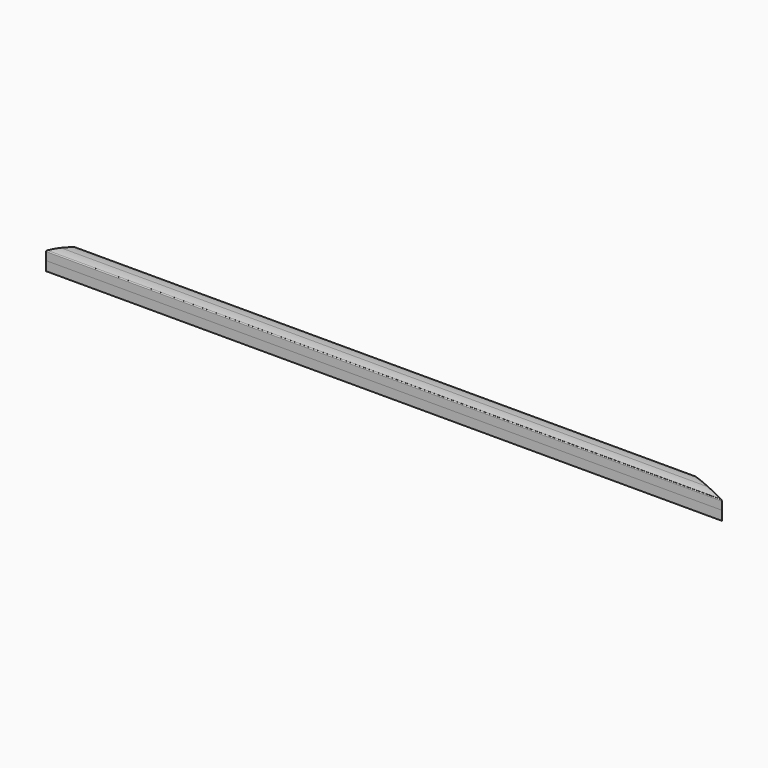
from build123d import *

# Parameters (mm, degrees)
F2_DEPTH      = 1000
F4_DEPTH      = 1000
F8_DEPTH      = 10.001
F8_DEPTH_BACK = 10.001


# Not quite as in the source:
# - ends of sketch curves that miss each other by under 0.0002 mm in the source are joined


with BuildPart() as f2:
    # F1 (on Right) → F2 (new body)
    with BuildSketch(Plane.YZ):
        with BuildLine():
            Line((0, -9), (0, -10))
            Line((0, -10), (10, -10))
            Line((10, -10), (10, -0.2))
            Line((10, -0.2), (9, -0.2))
            ThreePointArc((9, -0.2), (8.5, -0.7), (9, -1.2))
            ThreePointArc((9, -1.2), (9.5, -1.7), (9, -2.2))
            Line((9, -2.2), (9, -9))
            Line((9, -9), (0, -9))
        make_face()
    extrude(amount=F2_DEPTH)

    # F5: F2 across plane


with BuildPart() as f4:
    # F3 (on Right) → F4 (new body)
    with BuildSketch(Plane.YZ):
        with BuildLine():
            Line((9, -0.2), (10, -0.2))
            Line((10, -0.2), (10, 8.1663783152))
            ThreePointArc((10, 8.1663783152), (9.7693092582, 8.8052548802), (9.1836734694, 9.1493656277))
            ThreePointArc((9.1836734694, 9.1493656277), (4.6114920912, 9.7868872364), (0, 10))
            Line((0, 10), (0, 9))
            ThreePointArc((0, 9), (4.5192622493, 8.7911494917), (9, 8.1663783152))
            Line((9, 8.1663783152), (9, 0.8))
            ThreePointArc((9, 0.8), (7.5, -0.7), (9, -2.2))
            ThreePointArc((9, -2.2), (9.5, -1.7), (9, -1.2))
            ThreePointArc((9, -1.2), (8.5, -0.7), (9, -0.2))
        make_face()
    extrude(amount=F4_DEPTH)

    # F6: F4 across plane


with BuildPart() as f2_1:
    add(f2.part)
    add(f2.part.mirror(Plane.XZ))


with BuildPart() as f4_1:
    add(f4.part)
    add(f4.part.mirror(Plane.XZ))


with BuildPart() as f8_tool:
    # F7 (on Top) → F8 (new body, two sides)
    with BuildSketch(Plane.XY) as f8_sk:
        Polygon((0, 10), (0, 0), (0, -10), (15.0710810021, 10), align=None)
        Polygon((665.4979817736, 10), (710, -10), (1016.9613361359, -10), (1016.9613361359, 10), (709.9114895723, 10), align=None)
    extrude(amount=F8_DEPTH)
    extrude(f8_sk.sketch, amount=-F8_DEPTH_BACK)


with BuildPart() as f2_2:
    add(f2_1.part)

    # F8: cut by f8_tool
    add(f8_tool.part, mode=Mode.SUBTRACT)


with BuildPart() as f4_2:
    add(f4_1.part)

    # F8: cut by f8_tool
    add(f8_tool.part, mode=Mode.SUBTRACT)


solid = Compound([f2_2.part, f4_2.part])
